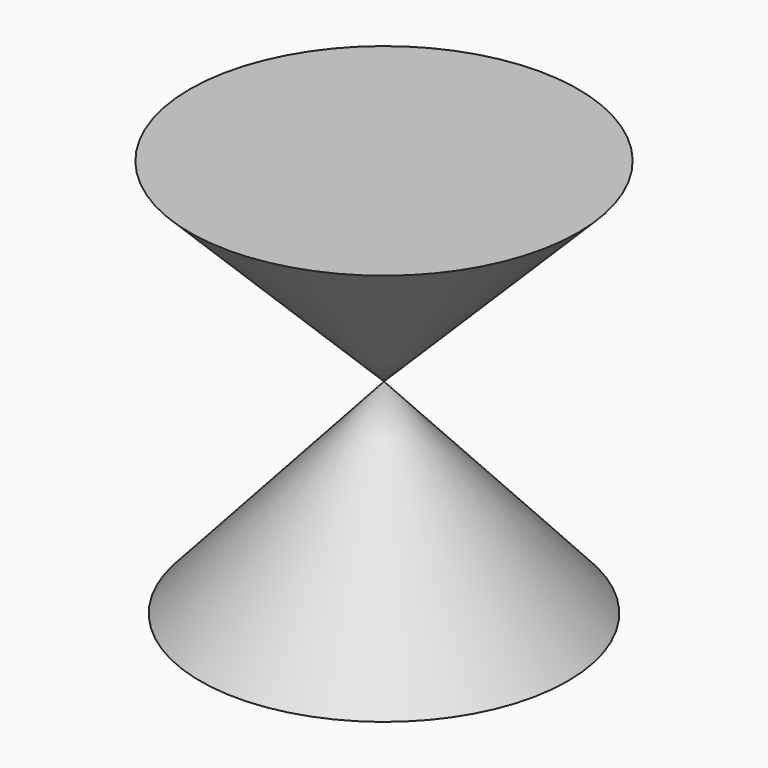
from build123d import *


# Not quite as in the source:
# - the program builds the solid bodies; features that only make, move or delete a surface that nothing else refers to are left out


with BuildPart() as f1:
    # F0 (on Front) → F1 (revolve)
    with BuildSketch(Plane.XZ):
        Polygon((-52.9157482088, -0.7591461658), (23.2842517912, 75.4408538342), (-52.9157482088, 75.4408538342), align=None)
    revolve(axis=Axis((-52.9157482088, 0, -2.7009313729), (0, 0, -1)))


with BuildPart() as f1b:
    # F0 (on Front) → F1, piece 2 (revolve)
    with BuildSketch(Plane.XZ):
        Polygon((19.1918224738, -80.8427165799), (-52.9157482088, -0.7591461658), (-52.9157482088, -80.8427165799), align=None)
    revolve(axis=Axis((-52.9157482088, 0, -2.7009313729), (0, 0, -1)))


solid = Compound([f1.part, f1b.part])
